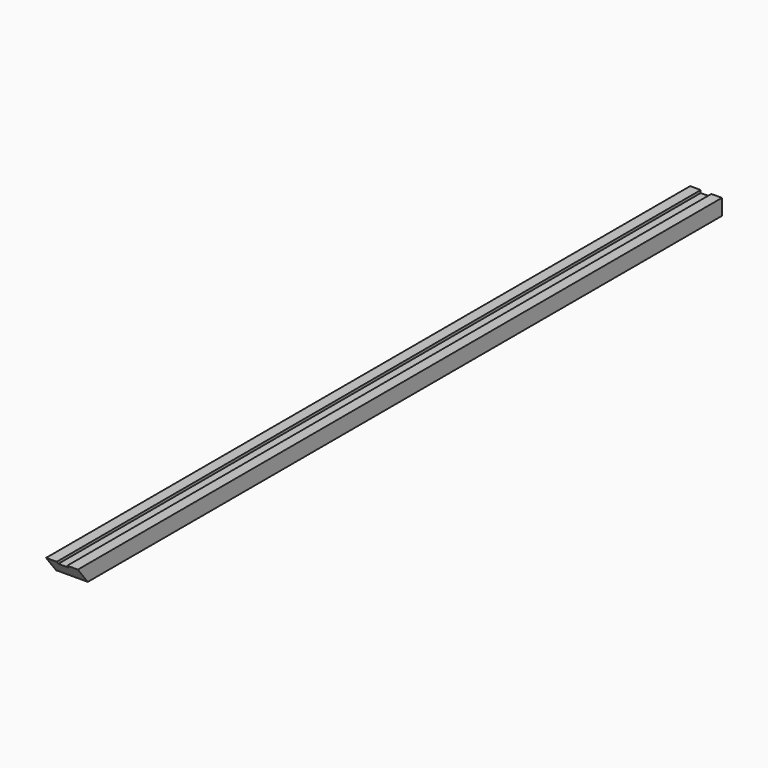
from build123d import *

# Parameters (mm, degrees)
F1_DEPTH    = 1930.4
F2_T1_DEPTH = 272.7606343602


# Not quite as in the source:
# - a fillet or chamfer that OpenCascade refuses, or shapes differently, is made with other operations: its cross-section is extruded or revolved along the edge and cut away or added


with BuildPart() as f1:
    # F0 (on Front) → F1 (new body)
    with BuildSketch(Plane.XZ):
        Polygon((0, 38.1), (0, 0), (76.2, 0), (76.2, 38.1), (50.8, 38.1), (50.8, 31.75), (25.4, 31.75), (25.4, 38.1), align=None)
    extrude(amount=F1_DEPTH)

    # F2: chamfer of 38.1 x 29.7669823699 on 1 edges, made by hand

    # F2_s2 → F2_t1 (cut)
    with BuildSketch(Plane.YZ.offset(-98.2803171801)):
        Polygon((-1900.6330176301, 0), (-1930.4, 38.1), (-1930.4, 0), align=None)
    extrude(amount=F2_T1_DEPTH, mode=Mode.SUBTRACT)


solid = f1.part
